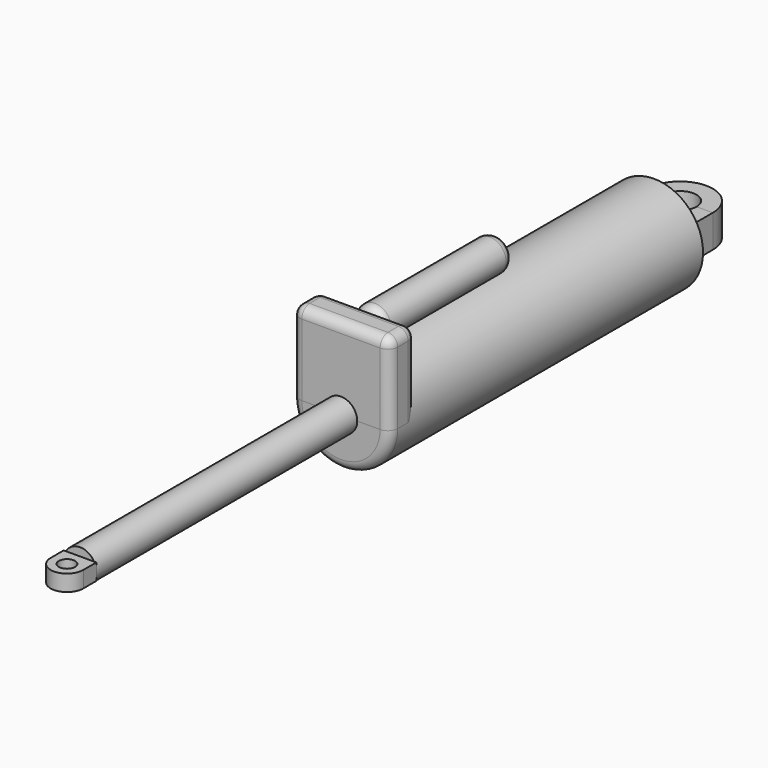
from build123d import *

# Parameters (mm, degrees)
F0_R      = 12.7
F1_DEPTH  = 254
F0_R_2    = 38.1
F2_DEPTH  = 304.8
F3_W      = 38.1
F3_H      = 63.5
F4_DEPTH  = 25.4
F5_R      = 12.7
F6_DEPTH  = 127
F7_DEPTH  = 304.8
F8_W      = 50.8
F8_H      = 25.4
F9_DEPTH  = 25.4
F11_DEPTH = 25.4
F13_D     = 25.4
F13_2_D   = 25.4
F14_R     = 7.62
F14_2_R   = 7.62
F14_3_R   = 7.62
F15_W     = 25.4
F15_H     = 6.3500005325
F16_DEPTH = 12.7
F18_DEPTH = 12.7
F20_D     = 12.7


# Not quite as in the source:
# - ends of sketch curves that miss each other by under 0.0002 mm in the source are joined


with BuildPart() as f1:
    # F0 (on Front) → F1 (new body)
    with BuildSketch(Plane.XZ):
        Circle(F0_R)
    extrude(amount=F1_DEPTH)


with BuildPart() as f2:
    # F0 (on Front) → F2 (new body)
    with BuildSketch(Plane.XZ):
        Circle(F0_R_2)
        Circle(F0_R, mode=Mode.SUBTRACT)
    extrude(amount=-F2_DEPTH)

    # F14#3
    f14_3_edges = [f2.edges().sort_by_distance(p)[0] for p in [
        (-38.1, 0, 0),
    ]]
    fillet(f14_3_edges, radius=F14_3_R)


with BuildPart() as f4:
    # F3 (on Front) → F4 (new body)
    with BuildSketch(Plane.XZ):
        with Locations((19.05, 31.75)):
            Rectangle(F3_W, F3_H)
        with Locations((-19.05, 31.75)):
            Rectangle(F3_W, F3_H)
    extrude(amount=-F4_DEPTH)

    # F14
    f14_edges = [f4.edges().sort_by_distance(p)[0] for p in [
        (38.1, 12.7, 63.5),
        (0, 25.4, 63.5),
        (-38.1, 12.7, 63.5),
        (0, 0, 63.5),
        (38.1, 25.4, 31.75),
        (38.1, 0, 31.75),
        (-38.1, 25.4, 31.75),
        (-38.1, 0, 31.75),
    ]]
    fillet(f14_edges, radius=F14_R)


with BuildPart() as f6:
    # F5 (on face) → F6 (new body)
    with BuildSketch(Plane(origin=(0, 25.4, 0), x_dir=(-1, 0, 0), z_dir=(0, 1, 0))):
        with Locations((0, 50.4958219826)):
            Circle(F5_R)
    extrude(amount=F6_DEPTH)

    # F14#2
    f14_2_edges = [f6.edges().sort_by_distance(p)[0] for p in [
        (12.7, 25.4, 50.495822),
        (12.7, 152.4, 50.495822),
    ]]
    fillet(f14_2_edges, radius=F14_2_R)


with BuildPart() as f7:
    # F7 (new): a face of the model
    f7_faces = [f1.part.faces().sort_by_distance(p)[0] for p in [
        (0, 0, 0),
    ]]
    extrude(f7_faces, amount=F7_DEPTH)


with BuildPart() as f9:
    # F8 (on face) → F9 (new body)
    with BuildSketch(Plane(origin=(0, 304.8, 0), x_dir=(-1, 0, 0), z_dir=(0, 1, 0))):
        Rectangle(F8_W, F8_H)
    extrude(amount=F9_DEPTH)

    # F13 (through all)
    with Locations(Plane.XY.offset(12.7)):
        with Locations((0, 330.2)):
            Hole(F13_D / 2)


with BuildPart() as f11:
    # F10 (on face) → F11 (new body)
    with BuildSketch(Plane.XY.offset(12.7)):
        with BuildLine():
            Line((-25.4, 330.2), (25.4, 330.2))
            ThreePointArc((25.4, 330.2), (0, 355.6), (-25.4, 330.2))
        make_face()
    extrude(amount=-F11_DEPTH)

    # F13#2 (through all)
    with Locations(Plane.XY.offset(12.7)):
        with Locations((0, 330.2)):
            Hole(F13_2_D / 2)


with BuildPart() as f1_1:
    add(f1.part)

    # F15 (on face) → F16 (join)
    with BuildSketch(Plane.XZ.offset(254)):
        Polygon((12.7, -6.35), (12.7, 0), (-12.7, -5.325e-07), (-12.7, -6.35), align=None)
        with Locations((0, 3.1749997337)):
            Rectangle(F15_W, F15_H)
    extrude(amount=F16_DEPTH)

    # F17 (on face) → F18 (join)
    with BuildSketch(Plane.XY.offset(6.35)):
        with BuildLine():
            Line((12.7, -266.7), (-12.7, -266.7))
            ThreePointArc((-12.7, -266.7), (0, -279.4), (12.7, -266.7))
        make_face()
    extrude(amount=-F18_DEPTH)

    # F20 (through all)
    with Locations(Plane.XY.offset(6.35)):
        with Locations((0, -266.7)):
            Hole(F20_D / 2)


solid = Compound([f2.part, f4.part, f6.part, f7.part, f9.part, f11.part, f1_1.part])
